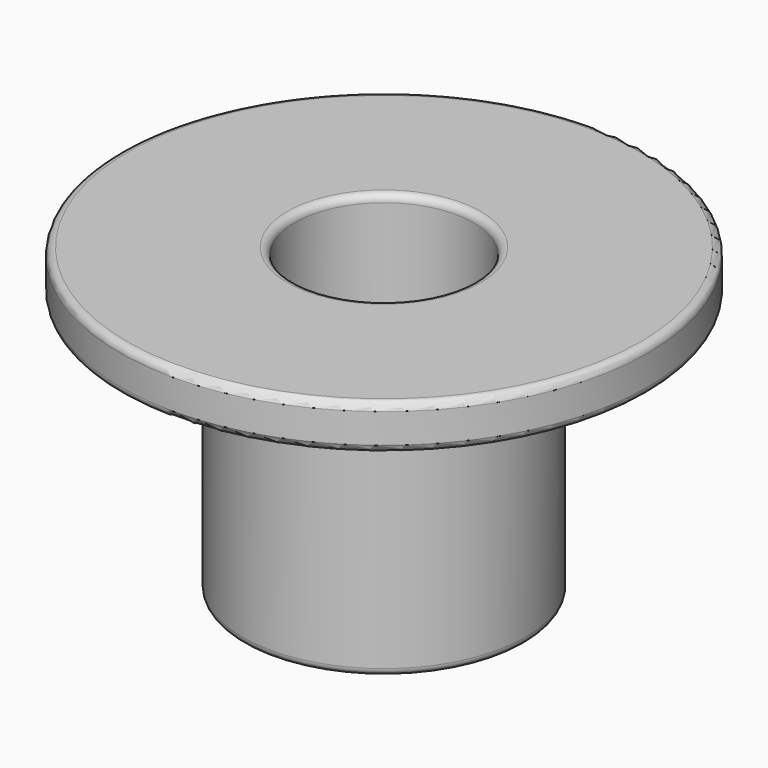
from build123d import *

# Parameters (mm, degrees)
F0_R     = 9.525
F0_R_2   = 6
F1_DEPTH = 17.5
F2_R     = 17.75
F2_R_2   = 6
F3_DEPTH = 3
F4_R     = 0.5


with BuildPart() as f1:
    # F0 (on Top) → F1 (new body)
    with BuildSketch(Plane.XY):
        Circle(F0_R)
        Circle(F0_R_2, mode=Mode.SUBTRACT)
    extrude(amount=-F1_DEPTH)

    # F2 (on Top) → F3 (join)
    with BuildSketch(Plane.XY):
        Circle(F2_R)
        Circle(F2_R_2, mode=Mode.SUBTRACT)
    extrude(amount=F3_DEPTH)

    # F4
    f4_edges = [f1.edges().sort_by_distance(p)[0] for p in [
        (-9.525, 0, -17.5),
        (-6, 0, -17.5),
        (-17.75, 0, 0),
        (-9.525, 0, 0),
        (-17.75, 0, 3),
        (-6, 0, 3),
    ]]
    fillet(f4_edges, radius=F4_R)


solid = f1.part
